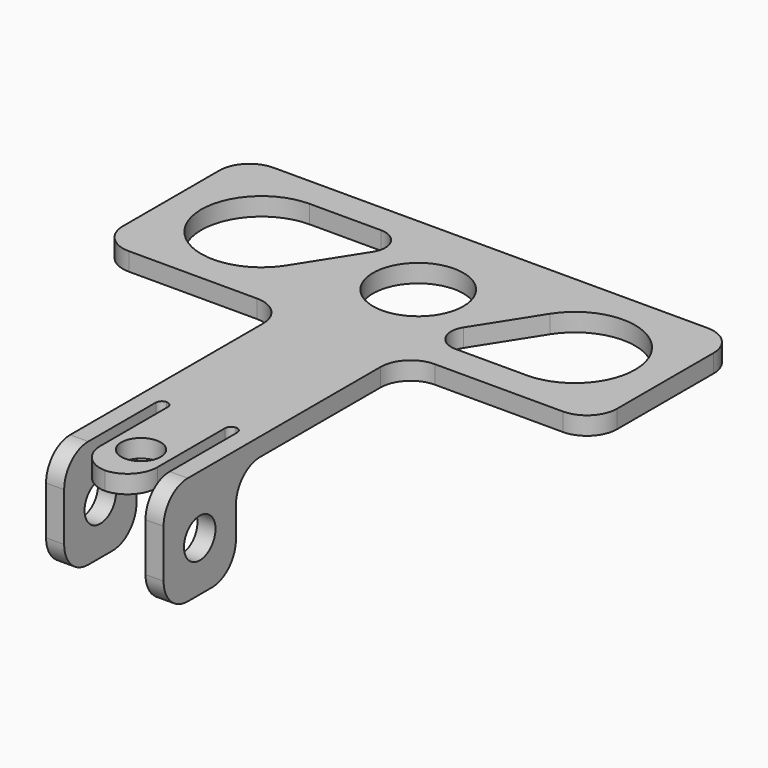
from build123d import *

# Parameters (mm, degrees)
F1_R         = 7.5
F1_R_2       = 3.2691742077
F2_DEPTH     = 3
F3_W         = 3
F3_H         = 15
F4_DEPTH     = 15
F5_R         = 3.2691742077
F6_DEPTH     = 50.751
F7_T1_DEPTH  = 3
F7_T3_DEPTH  = 3
F7_T5_DEPTH  = 3
F7_T7_DEPTH  = 28
F7_T9_DEPTH  = 15.5
F7_T11_DEPTH = 28
F7_T13_DEPTH = 28
F7_T15_DEPTH = 15.5
F8_R         = 0.99999


# Not quite as in the source:
# - a fillet or chamfer that OpenCascade refuses, or shapes differently, is made with other operations: its cross-section is extruded or revolved along the edge and cut away or added
# - a fillet or chamfer is up to 0.001 mm smaller than in the source, because OpenCascade refuses the exact size


with BuildPart() as f2:
    # F1 (on Top) → F2 (new body)
    with BuildSketch(Plane.XY):
        Polygon((41, 15), (-41, 15), (-41, -15), (-9.75, -15), (9.75, -15), (41, -15), align=None)
        with BuildLine():
            ThreePointArc((-17.5600507895, -5.3635116598), (-34.7645626416, -4.8148148148), (-26, 10))
            Line((-26, 10), (-14.1678404338, 10))
            ThreePointArc((-14.1678404338, 10), (-11.1002435092, 8.1851851852), (-11.2138582101, 4.6227709191))
            Line((-11.2138582101, 4.6227709191), (-17.5600507895, -5.3635116598))
        make_face(mode=Mode.SUBTRACT)
        Circle(F1_R, mode=Mode.SUBTRACT)
        with BuildLine():
            ThreePointArc((17.5600507895, 5.3635116598), (34.7645626416, 4.8148148148), (26, -10))
            Line((26, -10), (14.1678404338, -10))
            ThreePointArc((14.1678404338, -10), (11.1002435092, -8.1851851852), (11.2138582101, -4.6227709191))
            Line((11.2138582101, -4.6227709191), (17.5600507895, 5.3635116598))
        make_face(mode=Mode.SUBTRACT)
        Polygon((9.75, -15), (-9.75, -15), (-9.75, -65), (-6.75, -65), (-6.75, -45), (-4.75, -45), (-4.75, -65), (4.75, -65), (4.75, -45), (6.75, -45), (6.75, -65), (9.75, -65), align=None)
        with Locations((0, -57.5)):
            Circle(F1_R_2, mode=Mode.SUBTRACT)
    extrude(amount=F2_DEPTH)

    # F3 (on face) → F4 (join)
    with BuildSketch(Plane(origin=(0, 0, 0), x_dir=(1, 0, 0), z_dir=(0, 0, -1))):
        with Locations((8.25, 57.5)):
            Rectangle(F3_W, F3_H)
        with Locations((-8.25, 57.5)):
            Rectangle(F3_W, F3_H)
    extrude(amount=F4_DEPTH)

    # F5 (on face) → F6 (cut, through all)
    with BuildSketch(Plane.YZ.offset(9.75)):
        with Locations((-57.5, -6.75)):
            Circle(F5_R)
    extrude(amount=-F6_DEPTH, mode=Mode.SUBTRACT)

    # F7: fillet of radius 5 on 16 edges, made by hand

    # F7_s2 → F7_t1 (join)
    with BuildSketch(Plane.XY):
        with BuildLine():
            ThreePointArc((-14.75, -15), (-11.2144660941, -16.4644660941), (-9.75, -20))
            Line((-9.75, -20), (-9.75, -15))
            Line((-9.75, -15), (-14.75, -15))
        make_face()
        with BuildLine():
            ThreePointArc((14.75, -15), (11.2144660941, -16.4644660941), (9.75, -20))
            Line((9.75, -20), (9.75, -15))
            Line((9.75, -15), (14.75, -15))
        make_face()
    extrude(amount=F7_T1_DEPTH)

    # F7_s4 → F7_t3 (join)
    with BuildSketch(Plane.YZ.offset(6.75)):
        with BuildLine():
            ThreePointArc((-45, 0), (-48.5355339059, -1.4644660941), (-50, -5))
            Line((-50, -5), (-50, 0))
            Line((-50, 0), (-45, 0))
        make_face()
    extrude(amount=F7_T3_DEPTH)

    # F7_s6 → F7_t5 (join)
    with BuildSketch(Plane.YZ.offset(-9.75)):
        with BuildLine():
            ThreePointArc((-45, 0), (-48.5355339059, -1.4644660941), (-50, -5))
            Line((-50, -5), (-50, 0))
            Line((-50, 0), (-45, 0))
        make_face()
    extrude(amount=F7_T5_DEPTH)

    # F7_s8 → F7_t7 (cut)
    with BuildSketch(Plane.XY.offset(-12.5)):
        with BuildLine():
            ThreePointArc((-36, 15), (-39.5355339059, 13.5355339059), (-41, 10))
            Line((-41, 10), (-41, 15))
            Line((-41, 15), (-36, 15))
        make_face()
        with BuildLine():
            ThreePointArc((36, 15), (39.5355339059, 13.5355339059), (41, 10))
            Line((41, 10), (41, 15))
            Line((41, 15), (36, 15))
        make_face()
        with BuildLine():
            ThreePointArc((41, -10), (39.5355339059, -13.5355339059), (36, -15))
            Line((36, -15), (41, -15))
            Line((41, -15), (41, -10))
        make_face()
        with BuildLine():
            ThreePointArc((-41, -10), (-39.5355339059, -13.5355339059), (-36, -15))
            Line((-36, -15), (-41, -15))
            Line((-41, -15), (-41, -10))
        make_face()
        with BuildLine():
            ThreePointArc((4.75, -60), (3.2855339059, -63.5355339059), (-0.25, -65))
            Line((-0.25, -65), (4.75, -65))
            Line((4.75, -65), (4.75, -60))
        make_face()
        with BuildLine():
            ThreePointArc((0.25, -65), (-3.2855339059, -63.5355339059), (-4.75, -60))
            Line((-4.75, -60), (-4.75, -65))
            Line((-4.75, -65), (0.25, -65))
        make_face()
    extrude(amount=F7_T7_DEPTH, mode=Mode.SUBTRACT)

    # F7_s10 → F7_t9 (cut)
    with BuildSketch(Plane.YZ.offset(-22.25)):
        with BuildLine():
            ThreePointArc((-60, 3), (-63.5355339059, 1.5355339059), (-65, -2))
            Line((-65, -2), (-65, 3))
            Line((-65, 3), (-60, 3))
        make_face()
    extrude(amount=F7_T9_DEPTH, mode=Mode.SUBTRACT)

    # F7_s12 → F7_t11 (cut)
    with BuildSketch(Plane.YZ.offset(-22.25)):
        with BuildLine():
            ThreePointArc((-50, -10), (-51.4644660941, -13.5355339059), (-55, -15))
            Line((-55, -15), (-50, -15))
            Line((-50, -15), (-50, -10))
        make_face()
        with BuildLine():
            ThreePointArc((-65, -10), (-63.5355339059, -13.5355339059), (-60, -15))
            Line((-60, -15), (-65, -15))
            Line((-65, -15), (-65, -10))
        make_face()
    extrude(amount=F7_T11_DEPTH, mode=Mode.SUBTRACT)

    # F7_s14 → F7_t13 (cut)
    with BuildSketch(Plane.YZ.offset(-5.75)):
        with BuildLine():
            ThreePointArc((-55, -15), (-51.4644660941, -13.5355339059), (-50, -10))
            Line((-50, -10), (-50, -15))
            Line((-50, -15), (-55, -15))
        make_face()
        with BuildLine():
            ThreePointArc((-65, -10), (-63.5355339059, -13.5355339059), (-60, -15))
            Line((-60, -15), (-65, -15))
            Line((-65, -15), (-65, -10))
        make_face()
    extrude(amount=F7_T13_DEPTH, mode=Mode.SUBTRACT)

    # F7_s16 → F7_t15 (cut)
    with BuildSketch(Plane.YZ.offset(6.75)):
        with BuildLine():
            ThreePointArc((-60, 3), (-63.5355339059, 1.5355339059), (-65, -2))
            Line((-65, -2), (-65, 3))
            Line((-65, 3), (-60, 3))
        make_face()
    extrude(amount=F7_T15_DEPTH, mode=Mode.SUBTRACT)

    # F8 (radius 1 in the source; OpenCascade refuses exactly that, so slightly less here)
    f8_edges = [f2.edges().sort_by_distance(p)[0] for p in [
        (4.75, -45, 1.5),
        (6.75, -45, 1.5),
        (-4.75, -45, 1.5),
        (-6.75, -45, 1.5),
    ]]
    fillet(f8_edges, radius=F8_R)


solid = f2.part
